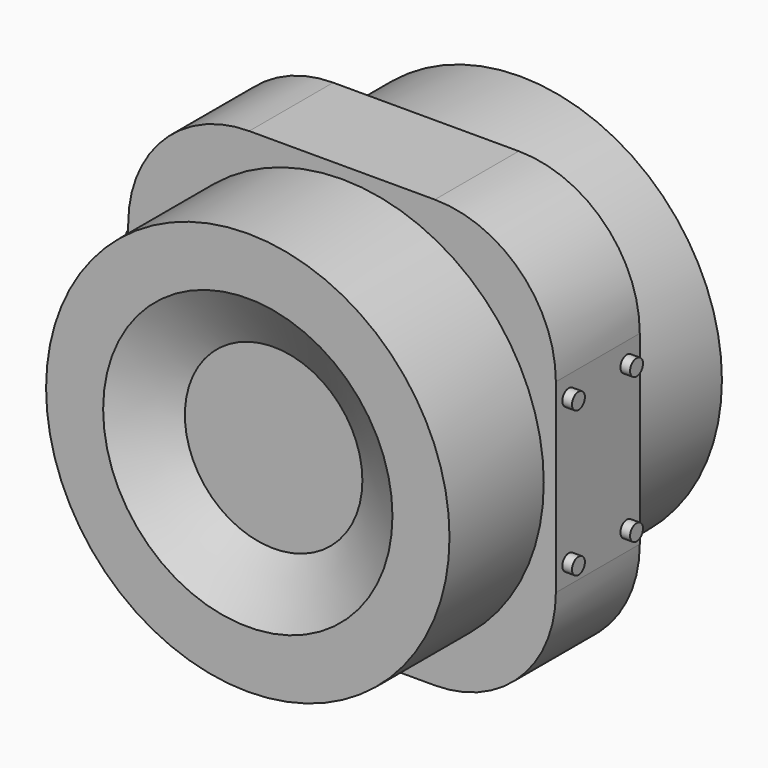
from build123d import *

# Parameters (mm, degrees)
F0_W          = 530
F0_H          = 530
F0_R          = 250
F1_DEPTH      = 65
F1_DEPTH_BACK = 65
F2_R          = 10
F3_DEPTH      = 12
F3_DEPTH_BACK = 542
F4_R          = 150
F0_R_2        = 110
F5_DEPTH      = 211
F5_DEPTH_BACK = 211
F6_DEPTH      = 171
F6_DEPTH_BACK = 171
F7_SIZE2      = 69.282022
F7_SIZE       = 39.99999
F8_SIZE2      = 69.282022
F8_SIZE       = 39.99999


# Not quite as in the source:
# - a fillet or chamfer is up to 0.001 mm smaller than in the source, because OpenCascade refuses the exact size


with BuildPart() as f1:
    # F0 (on Front) → F1 (new body, two sides)
    with BuildSketch(Plane.XZ) as f1_sk:
        Rectangle(F0_W, F0_H)
        Circle(F0_R, mode=Mode.SUBTRACT)
    extrude(amount=F1_DEPTH)
    extrude(f1_sk.sketch, amount=-F1_DEPTH_BACK)

    # F2 (on face) → F3 (join, two sides)
    with BuildSketch(Plane.YZ.offset(265)) as f3_sk:
        with Locations((-45, 90)):
            Circle(F2_R)
        with Locations((45, 90)):
            Circle(F2_R)
        with Locations((45, -90)):
            Circle(F2_R)
        with Locations((-45, -90)):
            Circle(F2_R)
    extrude(amount=F3_DEPTH)
    extrude(f3_sk.sketch, amount=-F3_DEPTH_BACK)

    # F4
    f4_edges = [f1.edges().sort_by_distance(p)[0] for p in [
        (265, 0, 265),
        (-265, 0, 265),
        (265, 0, -265),
        (-265, 0, -265),
    ]]
    fillet(f4_edges, radius=F4_R)

    # F0 (on Front) → F5 (join, two sides)
    with BuildSketch(Plane.XZ) as f5_sk:
        Circle(F0_R)
        Circle(F0_R_2, mode=Mode.SUBTRACT)
    extrude(amount=F5_DEPTH)
    extrude(f5_sk.sketch, amount=-F5_DEPTH_BACK)

    # F0 (on Front) → F6 (join, two sides)
    with BuildSketch(Plane.XZ) as f6_sk:
        Circle(F0_R_2)
    extrude(amount=F6_DEPTH)
    extrude(f6_sk.sketch, amount=-F6_DEPTH_BACK)

    # F7 (size 40 and 69.2820323028 in the source; OpenCascade refuses exactly that, so slightly less here)
    f7_edges = [f1.edges().sort_by_distance(p)[0] for p in [
        (-110, -211, 0),
    ]]
    f7_side = f1.faces().sort_by_distance((-110, -191, 0))[0]
    chamfer(f7_edges, length=F7_SIZE, length2=F7_SIZE2, reference=f7_side)

    # F8 (size 40 and 69.2820323028 in the source; OpenCascade refuses exactly that, so slightly less here)
    f8_edges = [f1.edges().sort_by_distance(p)[0] for p in [
        (-110, 211, 0),
    ]]
    f8_side = f1.faces().sort_by_distance((-110, 191, 0))[0]
    chamfer(f8_edges, length=F8_SIZE, length2=F8_SIZE2, reference=f8_side)


solid = f1.part
